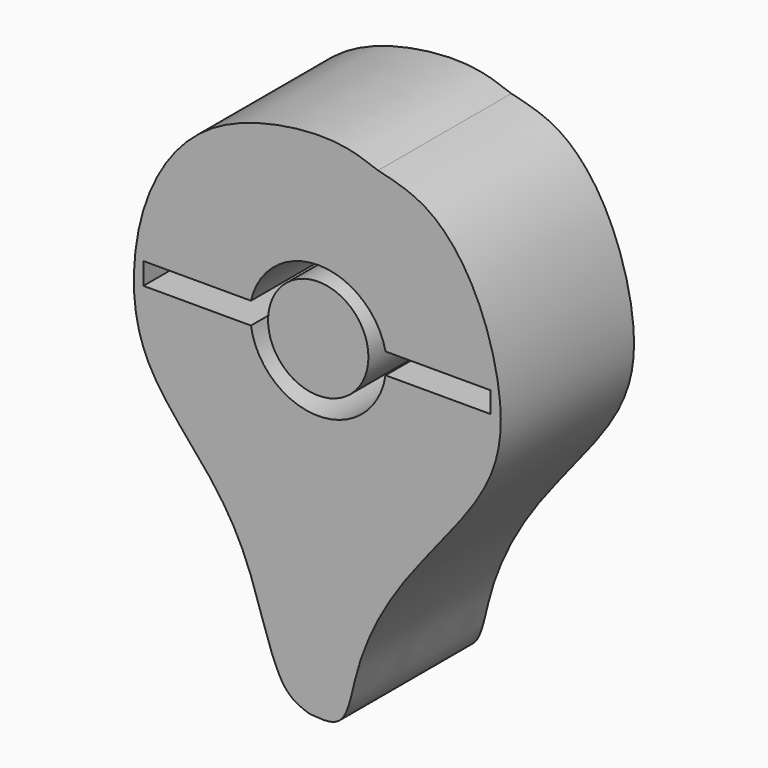
from build123d import *

# Parameters (mm, degrees)
F1_DEPTH = 25
F0_R     = 7.5303682966


with BuildPart() as f1:
    # F0 (on Front) → F1 (new body)
    with BuildSketch(Plane.XZ):
        with BuildLine():
            add(Edge.make_bspline(
                [(-11.9837475941, 41.112869978), (-14.0644761705, 41.886695284), (-19.2557934458, 43.8173520381), (-36.54394953, 41.0291184883), (-46.0001070067, 30.0422302578), (-49.2205246293, 17.5763953256), (-48.1474036096, 4.2025256185), (-37.2110825678, -6.8545940824), (-30.7871102029, -17.1470942803), (-27.2498735968, -32.3723669291), (-23.5453352756, -33.604638441), (-22.2246721387, -34.0439416468)],
                knots=[0, 0, 0, 0, 0.0878062704, 0.2190724025, 0.3395366578, 0.4535266556, 0.5685909876, 0.6925343203, 0.8090503071, 0.9319266806, 1, 1, 1, 1], degree=3))
            add(Edge.make_bspline(
                [(-22.2246721387, -34.0439416468), (-20.536529393, -34.1938452236), (-16.6236175005, -34.5413036894), (-15.4966338341, -25.0211298075), (-9.1613017918, -11.8441221828), (4.3688343274, 2.4843501308), (7.6345553851, 14.6093654307), (3.4271549286, 30.3095753231), (-4.1001211686, 39.2136412169), (-9.5248784444, 40.520508702), (-11.9837475941, 41.112869978)],
                knots=[0, 0, 0, 0, 0.0791722469, 0.1835117482, 0.329537453, 0.4941485798, 0.6239938761, 0.7719211757, 0.8966191561, 1, 1, 1, 1], degree=3))
        make_face()
        with BuildLine():
            Line((-31.0648977757, 14.4113143906), (-47.1998937428, 14.4113143906))
            Line((-47.1998937428, 14.4113143906), (-47.1998937428, 17.6907852292))
            Line((-47.1998937428, 17.6907852292), (-31.0648977757, 17.6907852292))
            ThreePointArc((-31.0648977757, 17.6907852292), (-20.9117375341, 25.6935033247), (-10.8633618802, 17.5596047193))
            Line((-10.8633618802, 17.5596047193), (4.8780944198, 17.5596047193))
            Line((4.8780944198, 17.5596047193), (4.8780944198, 14.4113143906))
            Line((4.8780944198, 14.4113143906), (-10.8633618802, 14.4113143906))
            ThreePointArc((-10.8633618802, 14.4113143906), (-20.9641298279, 5.7501454983), (-31.0648977757, 14.4113143906))
        make_face(mode=Mode.SUBTRACT)
    extrude(amount=F1_DEPTH)


with BuildPart() as f1b:
    # F0 (on Front) → F1, piece 2 (new body)
    with BuildSketch(Plane.XZ):
        with Locations((-20.9641298279, 15.9705535008)):
            Circle(F0_R)
    extrude(amount=F1_DEPTH)


solid = Compound([f1.part, f1b.part])
